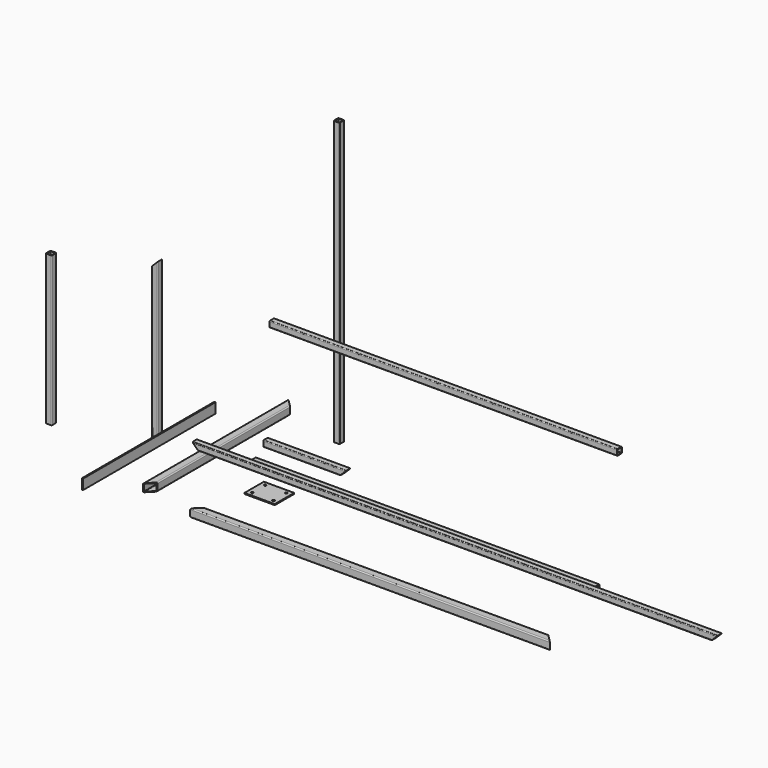
from build123d import *

# Parameters (mm, degrees)
F1_DEPTH  = 1700
F3_DEPTH  = 450
F5_DEPTH  = 1400
F7_DEPTH  = 1720
F8_W      = 150
F8_H      = 120
F8_R      = 5.5
F9_DEPTH  = 5
F11_DEPTH = 2600
F13_DEPTH = 800
F15_DEPTH = 410
F17_DEPTH = 740
F19_DEPTH = 842.3010538349
F21_DEPTH = 568.8829774985
F23_DEPTH = 403.101501895
F25_DEPTH = 1780
F1_FACE_W = 1700
F1_FACE_H = 30
F27_DEPTH = 103.6873894761
F28_DEPTH = 103.6873894761
F29_W     = 6
F29_H     = 50
F30_DEPTH = 820


with BuildPart() as f1:
    # F0 (on Right) → F1 (new body)
    with BuildSketch(Plane.YZ):
        with BuildLine():
            Line((-1.1402104422, 25.4200853229), (-31.1402104422, 25.4200853229))
            ThreePointArc((-31.1402104422, 25.4200853229), (-34.6757443482, 23.9556192289), (-36.1402104422, 20.4200853229))
            Line((-36.1402104422, 20.4200853229), (-36.1402104422, -9.5799146771))
            ThreePointArc((-36.1402104422, -9.5799146771), (-34.6757443482, -13.115448583), (-31.1402104422, -14.5799146771))
            Line((-31.1402104422, -14.5799146771), (-1.1402104422, -14.5799146771))
            ThreePointArc((-1.1402104422, -14.5799146771), (2.3953234637, -13.115448583), (3.8597895578, -9.5799146771))
            Line((3.8597895578, -9.5799146771), (3.8597895578, 20.4200853229))
            ThreePointArc((3.8597895578, 20.4200853229), (2.3953234637, 23.9556192289), (-1.1402104422, 25.4200853229))
        make_face()
        with BuildLine():
            ThreePointArc((-33.1402104422, 20.4200853229), (-32.5544240046, 21.8342988853), (-31.1402104422, 22.4200853229))
            Line((-31.1402104422, 22.4200853229), (-1.1402104422, 22.4200853229))
            ThreePointArc((-1.1402104422, 22.4200853229), (0.2740031201, 21.8342988853), (0.8597895578, 20.4200853229))
            Line((0.8597895578, 20.4200853229), (0.8597895578, -9.5799146771))
            ThreePointArc((0.8597895578, -9.5799146771), (0.2740031201, -10.9941282395), (-1.1402104422, -11.5799146771))
            Line((-1.1402104422, -11.5799146771), (-31.1402104422, -11.5799146771))
            ThreePointArc((-31.1402104422, -11.5799146771), (-32.5544240046, -10.9941282395), (-33.1402104422, -9.5799146771))
            Line((-33.1402104422, -9.5799146771), (-33.1402104422, 20.4200853229))
        make_face(mode=Mode.SUBTRACT)
    extrude(amount=F1_DEPTH)

    # F26 (on face) → F28 (cut, through all)
    with BuildSketch(Plane.XY.offset(31.6595588624)):
        Polygon((-198.3761233091, -450), (-158.3761233091, -450), (-158.3761233091, -410), align=None)
        Polygon((1780, -405.0449919701), (1780, -365.0449919701), (1740, -365.0449919701), align=None)
        Polygon((40, -365.0449919701), (0, -365.0449919701), (0, -405.0449919701), align=None)
        Polygon((-158.3761233091, 410), (-158.3761233091, 450), (-198.3761233091, 450), align=None)
    extrude(amount=-F28_DEPTH, mode=Mode.SUBTRACT)


with BuildPart() as f3:
    # F2 (on Front) → F3 (new body, symmetric)
    with BuildSketch(Plane.XZ):
        with BuildLine():
            Line((-163.3761233091, 31.6595588624), (-193.3761233091, 31.6595588624))
            ThreePointArc((-193.3761233091, 31.6595588624), (-196.9116572151, 30.1950927684), (-198.3761233091, 26.6595588624))
            Line((-198.3761233091, 26.6595588624), (-198.3761233091, -3.3404411376))
            ThreePointArc((-198.3761233091, -3.3404411376), (-196.9116572151, -6.8759750435), (-193.3761233091, -8.3404411376))
            Line((-193.3761233091, -8.3404411376), (-163.3761233091, -8.3404411376))
            ThreePointArc((-163.3761233091, -8.3404411376), (-159.8405894032, -6.8759750435), (-158.3761233091, -3.3404411376))
            Line((-158.3761233091, -3.3404411376), (-158.3761233091, 26.6595588624))
            ThreePointArc((-158.3761233091, 26.6595588624), (-159.8405894032, 30.1950927684), (-163.3761233091, 31.6595588624))
        make_face()
        with BuildLine():
            ThreePointArc((-195.3761233091, 26.6595588624), (-194.7903368715, 28.0737724248), (-193.3761233091, 28.6595588624))
            Line((-193.3761233091, 28.6595588624), (-163.3761233091, 28.6595588624))
            ThreePointArc((-163.3761233091, 28.6595588624), (-161.9619097468, 28.0737724248), (-161.3761233091, 26.6595588624))
            Line((-161.3761233091, 26.6595588624), (-161.3761233091, -3.3404411376))
            ThreePointArc((-161.3761233091, -3.3404411376), (-161.9619097468, -4.7546546999), (-163.3761233091, -5.3404411376))
            Line((-163.3761233091, -5.3404411376), (-193.3761233091, -5.3404411376))
            ThreePointArc((-193.3761233091, -5.3404411376), (-194.7903368715, -4.7546546999), (-195.3761233091, -3.3404411376))
            Line((-195.3761233091, -3.3404411376), (-195.3761233091, 26.6595588624))
        make_face(mode=Mode.SUBTRACT)
    extrude(amount=F3_DEPTH, both=True)


with BuildPart() as f5:
    # F4 (on Top) → F5 (new body)
    with BuildSketch(Plane.XY):
        with BuildLine():
            Line((149.1971788406, 357.0661640167), (127.1971788406, 357.0661640167))
            ThreePointArc((127.1971788406, 357.0661640167), (124.3687517159, 355.8945911415), (123.1971788406, 353.0661640167))
            Line((123.1971788406, 353.0661640167), (123.1971788406, 331.0661640167))
            ThreePointArc((123.1971788406, 331.0661640167), (124.3687517159, 328.237736892), (127.1971788406, 327.0661640167))
            Line((127.1971788406, 327.0661640167), (149.1971788406, 327.0661640167))
            ThreePointArc((149.1971788406, 327.0661640167), (152.0256059654, 328.237736892), (153.1971788406, 331.0661640167))
            Line((153.1971788406, 331.0661640167), (153.1971788406, 353.0661640167))
            ThreePointArc((153.1971788406, 353.0661640167), (152.0256059654, 355.8945911415), (149.1971788406, 357.0661640167))
        make_face()
        with BuildLine():
            ThreePointArc((126.1971788406, 353.0661640167), (126.4900720595, 353.7732707979), (127.1971788406, 354.0661640167))
            Line((127.1971788406, 354.0661640167), (149.1971788406, 354.0661640167))
            ThreePointArc((149.1971788406, 354.0661640167), (149.9042856218, 353.7732707979), (150.1971788406, 353.0661640167))
            Line((150.1971788406, 353.0661640167), (150.1971788406, 331.0661640167))
            ThreePointArc((150.1971788406, 331.0661640167), (149.9042856218, 330.3590572355), (149.1971788406, 330.0661640167))
            Line((149.1971788406, 330.0661640167), (127.1971788406, 330.0661640167))
            ThreePointArc((127.1971788406, 330.0661640167), (126.4900720595, 330.3590572355), (126.1971788406, 331.0661640167))
            Line((126.1971788406, 331.0661640167), (126.1971788406, 353.0661640167))
        make_face(mode=Mode.SUBTRACT)
    extrude(amount=F5_DEPTH)


with BuildPart() as f7:
    # F6 (on Right) → F7 (new body)
    with BuildSketch(Plane.YZ):
        with BuildLine():
            Line((111.6791767478, 585.846016407), (89.6791767478, 585.846016407))
            ThreePointArc((89.6791767478, 585.846016407), (86.8507496231, 584.6744435318), (85.6791767478, 581.846016407))
            Line((85.6791767478, 581.846016407), (85.6791767478, 559.846016407))
            ThreePointArc((85.6791767478, 559.846016407), (86.8507496231, 557.0175892823), (89.6791767478, 555.846016407))
            Line((89.6791767478, 555.846016407), (111.6791767478, 555.846016407))
            ThreePointArc((111.6791767478, 555.846016407), (114.5076038725, 557.0175892823), (115.6791767478, 559.846016407))
            Line((115.6791767478, 559.846016407), (115.6791767478, 581.846016407))
            ThreePointArc((115.6791767478, 581.846016407), (114.5076038725, 584.6744435318), (111.6791767478, 585.846016407))
        make_face()
        with BuildLine():
            ThreePointArc((88.6791767478, 581.846016407), (88.9720699666, 582.5531231882), (89.6791767478, 582.846016407))
            Line((89.6791767478, 582.846016407), (111.6791767478, 582.846016407))
            ThreePointArc((111.6791767478, 582.846016407), (112.386283529, 582.5531231882), (112.6791767478, 581.846016407))
            Line((112.6791767478, 581.846016407), (112.6791767478, 559.846016407))
            ThreePointArc((112.6791767478, 559.846016407), (112.386283529, 559.1389096258), (111.6791767478, 558.846016407))
            Line((111.6791767478, 558.846016407), (89.6791767478, 558.846016407))
            ThreePointArc((89.6791767478, 558.846016407), (88.9720699666, 559.1389096258), (88.6791767478, 559.846016407))
            Line((88.6791767478, 559.846016407), (88.6791767478, 581.846016407))
        make_face(mode=Mode.SUBTRACT)
    extrude(amount=F7_DEPTH)


with BuildPart() as f9:
    # F8 (on Top) → F9 (new body)
    with BuildSketch(Plane.XY):
        with Locations((201.7841267586, -167.9766052961)):
            Rectangle(F8_W, F8_H)
        with Locations((149.2841267586, -207.9766052961)):
            Circle(F8_R, mode=Mode.SUBTRACT)
        with Locations((254.2841267586, -207.9766052961)):
            Circle(F8_R, mode=Mode.SUBTRACT)
        with Locations((149.2841267586, -127.9766052961)):
            Circle(F8_R, mode=Mode.SUBTRACT)
        with Locations((254.2841267586, -127.9766052961)):
            Circle(F8_R, mode=Mode.SUBTRACT)
    extrude(amount=F9_DEPTH)


with BuildPart() as f11:
    # F10 (on Right) → F11 (new body)
    with BuildSketch(Plane.YZ):
        with BuildLine():
            Line((-366.3000538349, 252.8133386374), (-388.3000538349, 252.8133386374))
            ThreePointArc((-388.3000538349, 252.8133386374), (-391.1284809597, 251.6417657621), (-392.3000538349, 248.8133386374))
            Line((-392.3000538349, 248.8133386374), (-392.3000538349, 226.8133386374))
            ThreePointArc((-392.3000538349, 226.8133386374), (-391.1284809597, 223.9849115126), (-388.3000538349, 222.8133386374))
            Line((-388.3000538349, 222.8133386374), (-366.3000538349, 222.8133386374))
            ThreePointArc((-366.3000538349, 222.8133386374), (-363.4716267102, 223.9849115126), (-362.3000538349, 226.8133386374))
            Line((-362.3000538349, 226.8133386374), (-362.3000538349, 248.8133386374))
            ThreePointArc((-362.3000538349, 248.8133386374), (-363.4716267102, 251.6417657621), (-366.3000538349, 252.8133386374))
        make_face()
        with BuildLine():
            ThreePointArc((-389.3000538349, 248.8133386374), (-389.0071606161, 249.5204454185), (-388.3000538349, 249.8133386374))
            Line((-388.3000538349, 249.8133386374), (-366.3000538349, 249.8133386374))
            ThreePointArc((-366.3000538349, 249.8133386374), (-365.5929470537, 249.5204454185), (-365.3000538349, 248.8133386374))
            Line((-365.3000538349, 248.8133386374), (-365.3000538349, 226.8133386374))
            ThreePointArc((-365.3000538349, 226.8133386374), (-365.5929470537, 226.1062318562), (-366.3000538349, 225.8133386374))
            Line((-366.3000538349, 225.8133386374), (-388.3000538349, 225.8133386374))
            ThreePointArc((-388.3000538349, 225.8133386374), (-389.0071606161, 226.1062318562), (-389.3000538349, 226.8133386374))
            Line((-389.3000538349, 226.8133386374), (-389.3000538349, 248.8133386374))
        make_face(mode=Mode.SUBTRACT)
    extrude(amount=F11_DEPTH)

    # F18 (on face) → F19 (cut, through all)
    with BuildSketch(Plane.XZ.offset(392.3000538349)):
        Polygon((2570, 222.8133386374), (2600, 222.8133386374), (2600, 252.8133386374), align=None)
        Polygon((0, 252.8133386374), (0, 222.8133386374), (30, 222.8133386374), align=None)
    extrude(amount=-F19_DEPTH, mode=Mode.SUBTRACT)


with BuildPart() as f13:
    # F12 (on Top) → F13 (new body)
    with BuildSketch(Plane.XY):
        with BuildLine():
            Line((-393.7814011574, -88.8819774985), (-415.7814011574, -88.8819774985))
            ThreePointArc((-415.7814011574, -88.8819774985), (-418.6098282821, -90.0535503738), (-419.7814011574, -92.8819774985))
            Line((-419.7814011574, -92.8819774985), (-419.7814011574, -114.8819774985))
            ThreePointArc((-419.7814011574, -114.8819774985), (-418.6098282821, -117.7104046233), (-415.7814011574, -118.8819774985))
            Line((-415.7814011574, -118.8819774985), (-393.7814011574, -118.8819774985))
            ThreePointArc((-393.7814011574, -118.8819774985), (-390.9529740326, -117.7104046233), (-389.7814011574, -114.8819774985))
            Line((-389.7814011574, -114.8819774985), (-389.7814011574, -92.8819774985))
            ThreePointArc((-389.7814011574, -92.8819774985), (-390.9529740326, -90.0535503738), (-393.7814011574, -88.8819774985))
        make_face()
        with BuildLine():
            ThreePointArc((-416.7814011574, -92.8819774985), (-416.4885079386, -92.1748707173), (-415.7814011574, -91.8819774985))
            Line((-415.7814011574, -91.8819774985), (-393.7814011574, -91.8819774985))
            ThreePointArc((-393.7814011574, -91.8819774985), (-393.0742943762, -92.1748707173), (-392.7814011574, -92.8819774985))
            Line((-392.7814011574, -92.8819774985), (-392.7814011574, -114.8819774985))
            ThreePointArc((-392.7814011574, -114.8819774985), (-393.0742943762, -115.5890842797), (-393.7814011574, -115.8819774985))
            Line((-393.7814011574, -115.8819774985), (-415.7814011574, -115.8819774985))
            ThreePointArc((-415.7814011574, -115.8819774985), (-416.4885079386, -115.5890842797), (-416.7814011574, -114.8819774985))
            Line((-416.7814011574, -114.8819774985), (-416.7814011574, -92.8819774985))
        make_face(mode=Mode.SUBTRACT)
    extrude(amount=F13_DEPTH)

    # F20 (on face) → F21 (cut, through all)
    with BuildSketch(Plane.XZ.offset(118.8819774985)):
        Polygon((-389.7814011574, 800), (-419.7814011574, 800), (-419.7814011574, 770), align=None)
        Polygon((-419.7814011574, 30), (-419.7814011574, 0), (-389.7814011574, 0), align=None)
    extrude(amount=-F21_DEPTH, mode=Mode.SUBTRACT)


with BuildPart() as f15:
    # F14 (on Right) → F15 (new body)
    with BuildSketch(Plane.YZ):
        with BuildLine():
            Line((72.899498105, 81.1707744002), (50.899498105, 81.1707744002))
            ThreePointArc((50.899498105, 81.1707744002), (48.0710709803, 79.999201525), (46.899498105, 77.1707744002))
            Line((46.899498105, 77.1707744002), (46.899498105, 55.1707744002))
            ThreePointArc((46.899498105, 55.1707744002), (48.0710709803, 52.3423472755), (50.899498105, 51.1707744002))
            Line((50.899498105, 51.1707744002), (72.899498105, 51.1707744002))
            ThreePointArc((72.899498105, 51.1707744002), (75.7279252298, 52.3423472755), (76.899498105, 55.1707744002))
            Line((76.899498105, 55.1707744002), (76.899498105, 77.1707744002))
            ThreePointArc((76.899498105, 77.1707744002), (75.7279252298, 79.999201525), (72.899498105, 81.1707744002))
        make_face()
        with BuildLine():
            ThreePointArc((49.899498105, 77.1707744002), (50.1923913239, 77.8778811814), (50.899498105, 78.1707744002))
            Line((50.899498105, 78.1707744002), (72.899498105, 78.1707744002))
            ThreePointArc((72.899498105, 78.1707744002), (73.6066048862, 77.8778811814), (73.899498105, 77.1707744002))
            Line((73.899498105, 77.1707744002), (73.899498105, 55.1707744002))
            ThreePointArc((73.899498105, 55.1707744002), (73.6066048862, 54.463667619), (72.899498105, 54.1707744002))
            Line((72.899498105, 54.1707744002), (50.899498105, 54.1707744002))
            ThreePointArc((50.899498105, 54.1707744002), (50.1923913239, 54.463667619), (49.899498105, 55.1707744002))
            Line((49.899498105, 55.1707744002), (49.899498105, 77.1707744002))
        make_face(mode=Mode.SUBTRACT)
    extrude(amount=F15_DEPTH)

    # F22 (on face) → F23 (cut, through all)
    with BuildSketch(Plane.XZ.offset(-46.899498105)):
        Polygon((380, 51.1707744002), (410, 51.1707744002), (410, 81.1707744002), align=None)
    extrude(amount=-F23_DEPTH, mode=Mode.SUBTRACT)


with BuildPart() as f17:
    # F16 (on Top) → F17 (new body)
    with BuildSketch(Plane.XY):
        with BuildLine():
            Line((-817.5079598427, -215.4309904575), (-839.5079598427, -215.4309904575))
            ThreePointArc((-839.5079598427, -215.4309904575), (-842.3363869674, -216.6025633328), (-843.5079598427, -219.4309904575))
            Line((-843.5079598427, -219.4309904575), (-843.5079598427, -241.4309904575))
            ThreePointArc((-843.5079598427, -241.4309904575), (-842.3363869674, -244.2594175823), (-839.5079598427, -245.4309904575))
            Line((-839.5079598427, -245.4309904575), (-817.5079598427, -245.4309904575))
            ThreePointArc((-817.5079598427, -245.4309904575), (-814.6795327179, -244.2594175823), (-813.5079598427, -241.4309904575))
            Line((-813.5079598427, -241.4309904575), (-813.5079598427, -219.4309904575))
            ThreePointArc((-813.5079598427, -219.4309904575), (-814.6795327179, -216.6025633328), (-817.5079598427, -215.4309904575))
        make_face()
        with BuildLine():
            ThreePointArc((-840.5079598427, -219.4309904575), (-840.2150666239, -218.7238836763), (-839.5079598427, -218.4309904575))
            Line((-839.5079598427, -218.4309904575), (-817.5079598427, -218.4309904575))
            ThreePointArc((-817.5079598427, -218.4309904575), (-816.8008530615, -218.7238836763), (-816.5079598427, -219.4309904575))
            Line((-816.5079598427, -219.4309904575), (-816.5079598427, -241.4309904575))
            ThreePointArc((-816.5079598427, -241.4309904575), (-816.8008530615, -242.1380972387), (-817.5079598427, -242.4309904575))
            Line((-817.5079598427, -242.4309904575), (-839.5079598427, -242.4309904575))
            ThreePointArc((-839.5079598427, -242.4309904575), (-840.2150666239, -242.1380972387), (-840.5079598427, -241.4309904575))
            Line((-840.5079598427, -241.4309904575), (-840.5079598427, -219.4309904575))
        make_face(mode=Mode.SUBTRACT)
    extrude(amount=F17_DEPTH)


with BuildPart() as f25:
    # F24 (on Right) → F25 (new body)
    with BuildSketch(Plane.YZ):
        with BuildLine():
            Line((-370.0449919701, -32.0268306136), (-400.0449919701, -32.0268306136))
            ThreePointArc((-400.0449919701, -32.0268306136), (-403.580525876, -33.4912967077), (-405.0449919701, -37.0268306136))
            Line((-405.0449919701, -37.0268306136), (-405.0449919701, -67.0268306136))
            ThreePointArc((-405.0449919701, -67.0268306136), (-403.580525876, -70.5623645195), (-400.0449919701, -72.0268306136))
            Line((-400.0449919701, -72.0268306136), (-370.0449919701, -72.0268306136))
            ThreePointArc((-370.0449919701, -72.0268306136), (-366.5094580641, -70.5623645195), (-365.0449919701, -67.0268306136))
            Line((-365.0449919701, -67.0268306136), (-365.0449919701, -37.0268306136))
            ThreePointArc((-365.0449919701, -37.0268306136), (-366.5094580641, -33.4912967077), (-370.0449919701, -32.0268306136))
        make_face()
        with BuildLine():
            ThreePointArc((-402.0449919701, -37.0268306136), (-401.4592055324, -35.6126170512), (-400.0449919701, -35.0268306136))
            Line((-400.0449919701, -35.0268306136), (-370.0449919701, -35.0268306136))
            ThreePointArc((-370.0449919701, -35.0268306136), (-368.6307784077, -35.6126170512), (-368.0449919701, -37.0268306136))
            Line((-368.0449919701, -37.0268306136), (-368.0449919701, -67.0268306136))
            ThreePointArc((-368.0449919701, -67.0268306136), (-368.6307784077, -68.441044176), (-370.0449919701, -69.0268306136))
            Line((-370.0449919701, -69.0268306136), (-400.0449919701, -69.0268306136))
            ThreePointArc((-400.0449919701, -69.0268306136), (-401.4592055324, -68.441044176), (-402.0449919701, -67.0268306136))
            Line((-402.0449919701, -67.0268306136), (-402.0449919701, -37.0268306136))
        make_face(mode=Mode.SUBTRACT)
    extrude(amount=F25_DEPTH)


with BuildPart() as f27_tool:
    # F26 (on face) + F1_face (on face) → F27 (new body, through all)
    with BuildSketch(Plane.XY.offset(31.6595588624)):
        Polygon((-198.3761233091, -450), (-158.3761233091, -450), (-158.3761233091, -410), align=None)
        Polygon((1780, -405.0449919701), (1780, -365.0449919701), (1740, -365.0449919701), align=None)
        Polygon((40, -365.0449919701), (0, -365.0449919701), (0, -405.0449919701), align=None)
        Polygon((-158.3761233091, 410), (-158.3761233091, 450), (-198.3761233091, 450), align=None)
    with BuildSketch(Plane(origin=(850, -16.1402104422, 25.4200853229), x_dir=(1, 0, 0), z_dir=(0, 0, 1))):
        Rectangle(F1_FACE_W, F1_FACE_H)
    extrude(amount=-F27_DEPTH)


with BuildPart() as f3_1:
    add(f3.part)

    # F27: cut by f27_tool
    add(f27_tool.part, mode=Mode.SUBTRACT)


with BuildPart() as f25_1:
    add(f25.part)

    # F27: cut by f27_tool
    add(f27_tool.part, mode=Mode.SUBTRACT)


with BuildPart() as f30:
    # F29 (on Front) → F30 (new body)
    with BuildSketch(Plane.XZ):
        with Locations((-201.9698069223, 176.4751300216)):
            Rectangle(F29_W, F29_H)
    extrude(amount=F30_DEPTH)


solid = Compound([f1.part, f5.part, f7.part, f9.part, f11.part, f13.part, f15.part, f17.part, f3_1.part, f25_1.part, f30.part])
